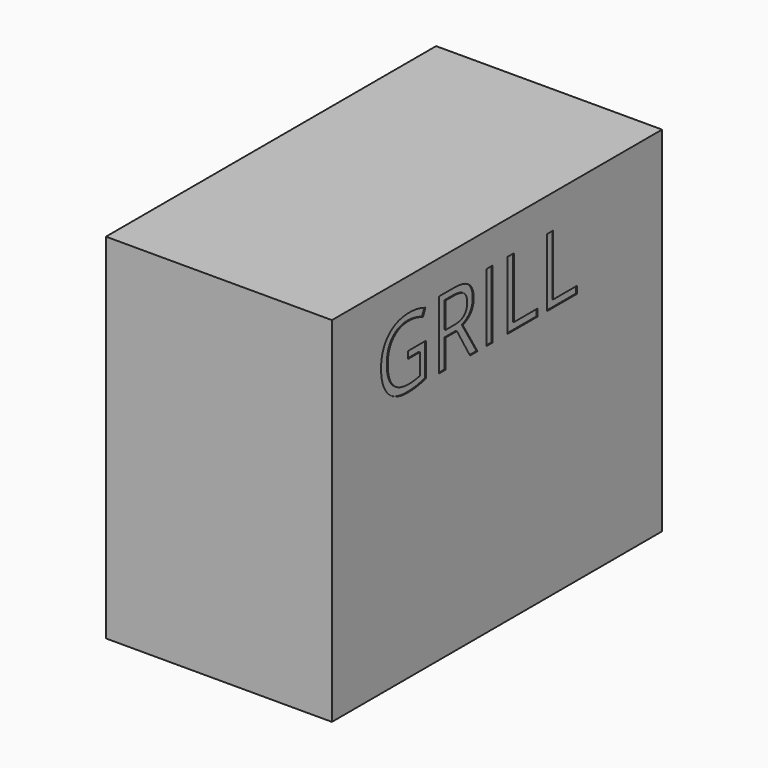
from build123d import *

# Parameters (mm, degrees)
F0_W         = 230
F0_H         = 420
F1_DEPTH     = 360
F2_TEXT_SIZE = 96.7575444116
F3_DEPTH     = 1


# Not quite as in the source:
# - Text() gives the source's letters only with a copy of the font that has no kerning and outlines rounded to 1/6400 em; it was checked with that copy


with BuildPart() as f1:
    # F0 (on Top) → F1 (new body)
    with BuildSketch(Plane.XY):
        Rectangle(F0_W, F0_H)
    extrude(amount=F1_DEPTH)

    # F2 (on face) → F3 (cut)
    with BuildSketch(Plane.YZ.offset(115)):
        with Locations((-153.4032672644, 256.7991316319)):
            Text('GRILL', F2_TEXT_SIZE, font='Open Sans', text_align=(TextAlign.LEFT, TextAlign.BOTTOM))
    extrude(amount=-F3_DEPTH, mode=Mode.SUBTRACT)


solid = f1.part
